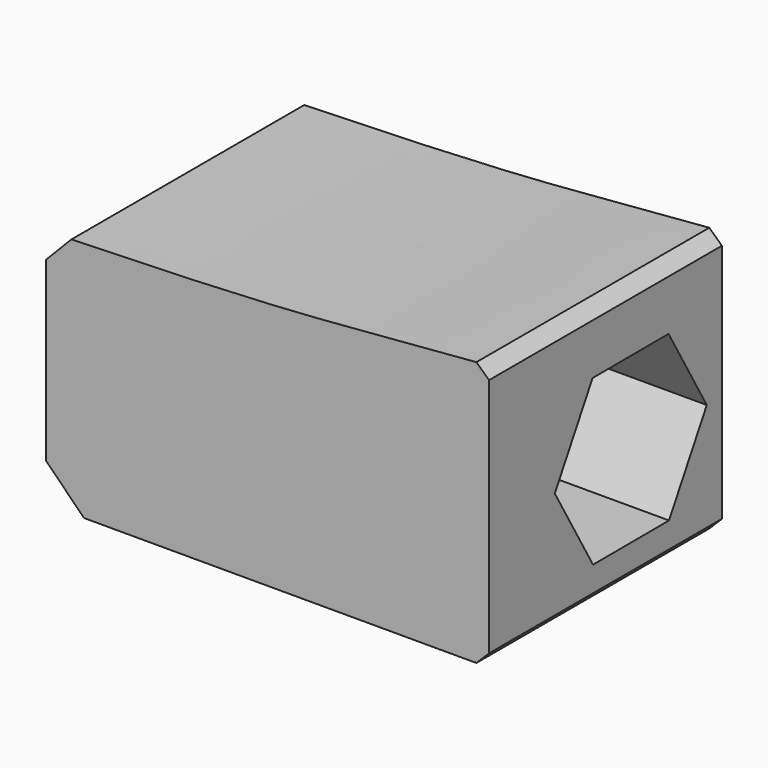
from build123d import *

# Parameters (mm, degrees)
F1_DEPTH    = 23
F2_R        = 4
F3_DEPTH    = 35.0010001
F5_DEPTH    = 32
F6_SIZE     = 1
F7_T1_DEPTH = 28.1474867513
F8_T1_DEPTH = 33.2835617863
F9_SIZE     = 3


# Not quite as in the source:
# - a fillet or chamfer that OpenCascade refuses, or shapes differently, is made with other operations: its cross-section is extruded or revolved along the edge and cut away or added


with BuildPart() as f1:
    # F0 (on Front) → F1 (new body)
    with BuildSketch(Plane.XZ):
        with BuildLine():
            Line((-35, 0), (0, 0))
            Line((0, 0), (0, 21))
            add(Edge.make_bspline(
                [(-35, 19), (-12.9749150947, 19.5710677654), (-12.9749150947, 20.0476832688), (0, 21)],
                knots=[0, 0, 0, 0, 35.0570962859, 35.0570962859, 35.0570962859, 35.0570962859], degree=3))
            Line((-35, 19), (-35, 0))
        make_face()
    extrude(amount=F1_DEPTH)

    # F2 (on Right) → F3 (cut, through all)
    with BuildSketch(Plane.YZ):
        with Locations((-9, 9.5)):
            Circle(F2_R)
    extrude(amount=-F3_DEPTH, mode=Mode.SUBTRACT)

    # F4 (on Right) → F5 (cut)
    with BuildSketch(Plane.YZ):
        Polygon((-5.225094273, 3.0128264948), (-1.4944900823, 9.5255775039), (-5.2693958093, 16.012751009), (-12.774905727, 15.9871735052), (-16.5055099177, 9.4744224961), (-12.7306041907, 2.987248991), align=None)
    extrude(amount=-F5_DEPTH, mode=Mode.SUBTRACT)

    # F6
    f6_edges = [f1.edges().sort_by_distance(p)[0] for p in [
        (0, -11.5, 0),
    ]]
    chamfer(f6_edges, length=F6_SIZE)

    # F7: chamfer of 1 on 1 edges, made by hand

    # F7_s2 → F7_t1 (cut)
    with BuildSketch(Plane.XZ.offset(-2.5737433757)):
        with BuildLine():
            Line((0.0293272632, 19.9718445491), (-1.0284200625, 20.9529152979))
            Line((-1.0284200625, 20.9529152979), (-1.0299222717, 20.9728588023))
            ThreePointArc((-1.0299222717, 20.9728588023), (-0.5146246013, 20.9820315927), (-0.0014639972, 21.0199463458))
            Line((-0.0014639972, 21.0199463458), (0.02, 21))
            ThreePointArc((0.02, 21), (0.02, 20.4859222745), (0.0493272632, 19.9718445491))
            Line((0.0493272632, 19.9718445491), (0.0293272632, 19.9718445491))
        make_face()
    extrude(amount=F7_T1_DEPTH, mode=Mode.SUBTRACT)

    # F8: chamfer of 2 on 1 edges, made by hand

    # F8_s2 → F8_t1 (cut)
    with BuildSketch(Plane.XZ.offset(-5.1417808931)):
        with BuildLine():
            Line((-35.0557899395, 16.944044455), (-32.9477944744, 19.1104787201))
            Line((-32.9477944744, 19.1104787201), (-32.9488880075, 19.1504637697))
            ThreePointArc((-32.9488880075, 19.1504637697), (-33.974209491, 19.0669652644), (-35.001036774, 19.0399865615))
            Line((-35.001036774, 19.0399865615), (-35.04, 19))
            ThreePointArc((-35.04, 19), (-35.04, 17.9720222275), (-35.0957899395, 16.944044455))
            Line((-35.0957899395, 16.944044455), (-35.0557899395, 16.944044455))
        make_face()
    extrude(amount=F8_T1_DEPTH, mode=Mode.SUBTRACT)

    # F9
    f9_edges = [f1.edges().sort_by_distance(p)[0] for p in [
        (-35, -11.5, 0),
    ]]
    chamfer(f9_edges, length=F9_SIZE)


solid = f1.part
